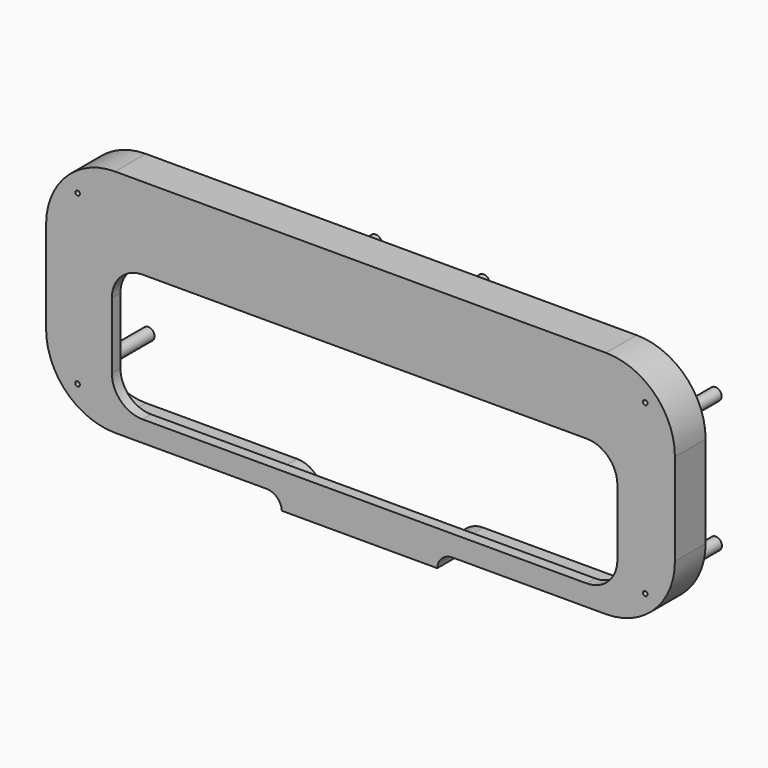
from build123d import *

# Parameters (mm, degrees)
F0_W           = 410
F0_H           = 150
F1_DEPTH       = 5
F1_DEPTH_BACK  = 20
F2_R           = 45
F3_R           = 45
F4_R           = 45
F5_W           = 101.2708619237
F5_H           = 20.8901241422
F6_DEPTH       = 5
F6_DEPTH_BACK  = 20
F7_T1_DEPTH    = 25
F8_T1_DEPTH    = 25
F10_T          = -7
F12_R          = 4
F13_DEPTH      = 55.5
F14_W          = 329.6116441488
F14_H          = 83.0728560686
F15_DEPTH      = 25
F15_DEPTH_BACK = 25
F16_R          = 20
F20_D          = 3
F20_DEPTH      = 20
F20_TIP        = 0.9012909285


# Not quite as in the source:
# - a fillet or chamfer that OpenCascade refuses, or shapes differently, is made with other operations: its cross-section is extruded or revolved along the edge and cut away or added


with BuildPart() as f1:
    # F0 (on Front) → F1 (new body, two sides)
    with BuildSketch(Plane.XZ) as f1_sk:
        Rectangle(F0_W, F0_H)
    extrude(amount=F1_DEPTH)
    extrude(f1_sk.sketch, amount=-F1_DEPTH_BACK)

    # F2
    f2_edges = [f1.edges().sort_by_distance(p)[0] for p in [
        (-205, 7.5, 75),
        (-205, 7.5, -75),
    ]]
    fillet(f2_edges, radius=F2_R)

    # F3
    f3_edges = [f1.edges().sort_by_distance(p)[0] for p in [
        (205, 7.5, 75),
    ]]
    fillet(f3_edges, radius=F3_R)

    # F4
    f4_edges = [f1.edges().sort_by_distance(p)[0] for p in [
        (205, 7.5, -75),
    ]]
    fillet(f4_edges, radius=F4_R)

    # F5 (on Front) → F6 (join, two sides)
    with BuildSketch(Plane.XZ) as f6_sk:
        with Locations((-0.6414987147, -73.9290080965)):
            Rectangle(F5_W, F5_H)
    extrude(amount=F6_DEPTH)
    extrude(f6_sk.sketch, amount=-F6_DEPTH_BACK)

    # F7: fillet of radius 10 on 1 edges, made by hand

    # F7_s2 → F7_t1 (join)
    with BuildSketch(Plane.XZ.offset(-20)):
        with BuildLine():
            ThreePointArc((-61.2573210439, -75), (-54.4111286103, -77.7109912085), (-51.2769296765, -84.3740701675))
            Line((-51.2769296765, -84.3740701675), (-51.2769296765, -75))
            Line((-51.2769296765, -75), (-61.2573210439, -75))
        make_face()
    extrude(amount=F7_T1_DEPTH)

    # F8: fillet of radius 10 on 1 edges, made by hand

    # F8_s2 → F8_t1 (join)
    with BuildSketch(Plane.XZ.offset(-20)):
        with BuildLine():
            ThreePointArc((49.9939322472, -84.3740701675), (53.1281311809, -77.7109912085), (59.9743236145, -75))
            Line((59.9743236145, -75), (49.9939322472, -75))
            Line((49.9939322472, -75), (49.9939322472, -84.3740701675))
        make_face()
    extrude(amount=F8_T1_DEPTH)

    # F10
    f10_openings = [f1.faces().sort_by_distance(p)[0] for p in [
        (-0.010473, 20, -1.299239),
    ]]
    offset(amount=F10_T, openings=f10_openings)

    # F12 (on offset) → F13 (join)
    with BuildSketch(Plane.XZ.offset(3)):
        with Locations((-184.3019276857, 36.01404652)):
            Circle(F12_R)
        with Locations((-184.2796504498, -49.4647398591)):
            Circle(F12_R)
        with Locations((-36.0691249371, 51.8314018846)):
            Circle(F12_R)
        with Locations((-49.5743155479, 31.3860401511)):
            Circle(F12_R)
        with Locations((34.2704169452, 51.8314018846)):
            Circle(F12_R)
        with Locations((49.4637563825, 31.7611843348)):
            Circle(F12_R)
        with Locations((185.4535341263, 36.2629145384)):
            Circle(F12_R)
        with Locations((185.6411099434, -49.4575425982)):
            Circle(F12_R)
    extrude(amount=-F13_DEPTH)

    # F14 (on face) → F15 (cut, two sides)
    with BuildSketch(Plane.XZ) as f15_sk:
        with Locations((2.6797705796, -19.8723953217)):
            Rectangle(F14_W, F14_H)
    extrude(amount=F15_DEPTH, mode=Mode.SUBTRACT)
    extrude(f15_sk.sketch, amount=-F15_DEPTH_BACK, mode=Mode.SUBTRACT)

    # F16
    f16_edges = [f1.edges().sort_by_distance(p)[0] for p in [
        (-162.126051, -1.5, 21.664033),
        (167.485593, -1.5, 21.664033),
        (167.485593, -1.5, -61.408823),
        (-162.126051, -1.5, -61.408823),
    ]]
    fillet(f16_edges, radius=F16_R)

    # F20
    with Locations(Plane.XZ.offset(5)):
        with Locations((-184.4574809074, 54.7145232558), (-184.4574809074, -54.8582747579), (185.6484860182, -54.8582747579), (185.6484860182, 54.7145232558)):
            Hole(F20_D / 2, depth=F20_DEPTH)
            with Locations((0, 0, -(F20_DEPTH + F20_TIP / 2))):  # 118° drill point
                Cone(0, F20_D / 2, F20_TIP, mode=Mode.SUBTRACT)


solid = f1.part
